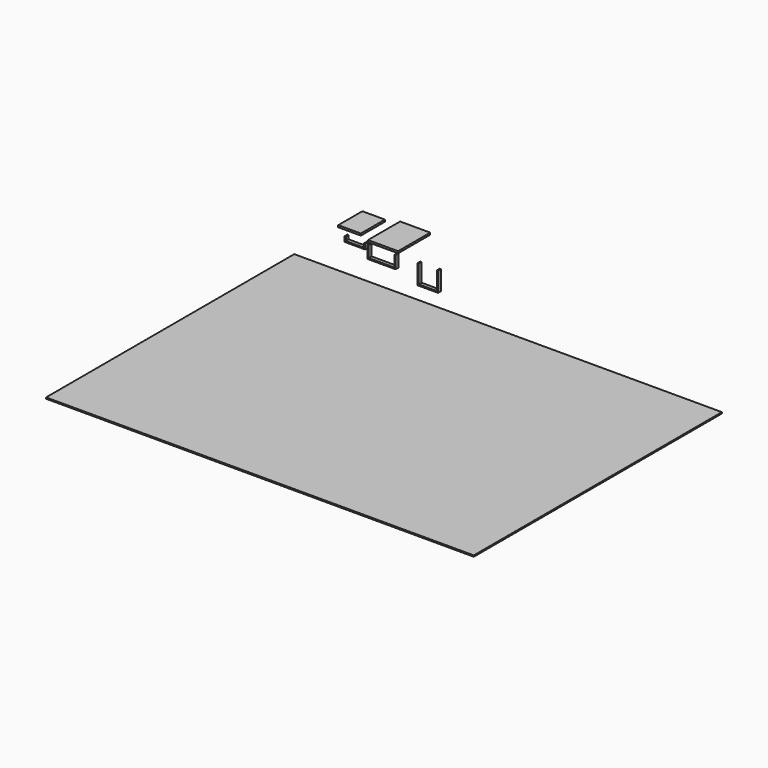
from build123d import *

# Parameters (mm, degrees)
F0_W      = 600
F0_H      = 800
F1_DEPTH  = 38
F3_DEPTH  = 70
F5_DEPTH  = 70
F9_DEPTH  = 70
F10_W     = 450
F10_H     = 600
F11_DEPTH = 38
F12_W     = 8515.9688591957
F12_H     = 6176.4018535614
F13_DEPTH = 25


# Not quite as in the source:
# - a feature of the source that left no trace in its solid (it failed there, or was rolled back) is left out


with BuildPart() as f1:
    # F0 (on Top) → F1 (new body)
    with BuildSketch(Plane.XY):
        with Locations((300, 400)):
            Rectangle(F0_W, F0_H)
    extrude(amount=F1_DEPTH)


with BuildPart() as f3:
    # F2 (on Front) → F3 (new body)
    with BuildSketch(Plane.XZ):
        Polygon((71.2579559533, 0), (46.2579559533, 0), (46.2579559533, -250), (606.2579559533, -250), (606.2579559533, 0), (581.2579559533, 0), (581.2579559533, -225), (71.2579559533, -225), align=None)
    extrude(amount=F3_DEPTH)


with BuildPart() as f5:
    # F4 (on Front) → F5 (new body)
    with BuildSketch(Plane.XZ):
        Polygon((0, -100), (0, 0), (-25, 0), (-25, -75), (-385, -75), (-385, 0), (-410, 0), (-410, -100), align=None)
    extrude(amount=F5_DEPTH)


with BuildPart() as f9:
    # F8 (on Front) → F9 (new body)
    with BuildSketch(Plane.XZ):
        Polygon((1067.0620972831, 0), (1042.0620972831, 0), (1042.0620972831, -388), (1452.0620972831, -388), (1452.0620972831, 0), (1427.0620972831, 0), (1427.0620972831, -363), (1067.0620972831, -363), align=None)
    extrude(amount=F9_DEPTH)


with BuildPart() as f11:
    # F10 (on Top) → F11 (new body)
    with BuildSketch(Plane.XY):
        with Locations((-449.1596068184, 402.8104767203)):
            Rectangle(F10_W, F10_H)
    extrude(amount=F11_DEPTH)


with BuildPart() as f13:
    # F12 (on Top) → F13 (new body)
    with BuildSketch(Plane.XY):
        with Locations((3643.9969241619, -4155.7756662369)):
            Rectangle(F12_W, F12_H)
    extrude(amount=F13_DEPTH)


solid = Compound([f1.part, f3.part, f5.part, f9.part, f11.part, f13.part])
